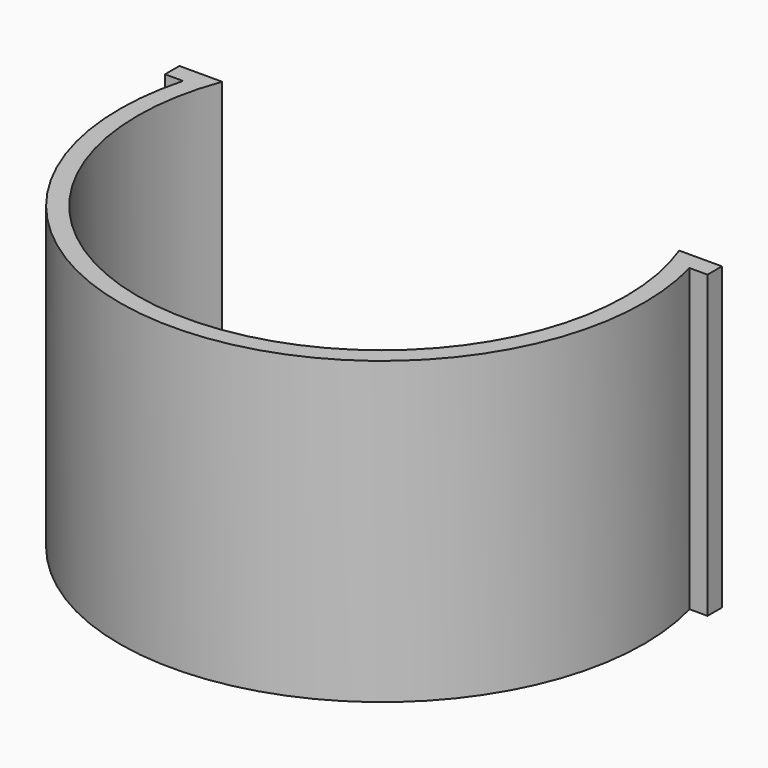
from build123d import *

# Parameters (mm, degrees)
F1_DEPTH = 250


# Not quite as in the source:
# - a feature names something its author has since deleted; it is built from what else it names


with BuildPart() as f1:
    # F0 (on Top) → F1 (new body)
    with BuildSketch(Plane.XY):
        with BuildLine():
            Line((-225.7312981026, 56.6), (-210.7312981026, 56.6))
            ThreePointArc((-210.7312981026, 56.6), (-208.5596069481, 64.1414869616), (-206.1181214741, 71.6))
            Line((-206.1181214741, 71.6), (-225.7312981026, 71.6))
            Line((-225.7312981026, 71.6), (-225.7312981026, 56.6))
        make_face()
        with BuildLine():
            ThreePointArc((206.1181214741, 71.6), (208.5596069481, 64.1414869616), (210.7312981026, 56.6))
            Line((210.7312981026, 56.6), (225.7312981026, 56.6))
            Line((225.7312981026, 56.6), (225.7312981026, 71.6))
            Line((225.7312981026, 71.6), (206.1181214741, 71.6))
        make_face()
        with BuildLine():
            ThreePointArc((-210.7312981026, 56.6), (-28.5453214557, -216.3247665502), (218.2, 0))
            ThreePointArc((218.2, 0), (216.3247665502, 28.5453214557), (210.7312981026, 56.6))
            ThreePointArc((210.7312981026, 56.6), (208.5596069481, 64.1414869616), (206.1181214741, 71.6))
            Line((206.1181214741, 71.6), (190.1675051106, 71.6))
            ThreePointArc((190.1675051106, 71.6), (199.9153283749, 36.3882052424), (203.2, 0))
            ThreePointArc((203.2, 0), (-36.3882052424, -199.9153283749), (-190.1675051106, 71.6))
            Line((-190.1675051106, 71.6), (-206.1181214741, 71.6))
            ThreePointArc((-206.1181214741, 71.6), (-208.5596069481, 64.1414869616), (-210.7312981026, 56.6))
        make_face()
    extrude(amount=F1_DEPTH)


solid = f1.part
